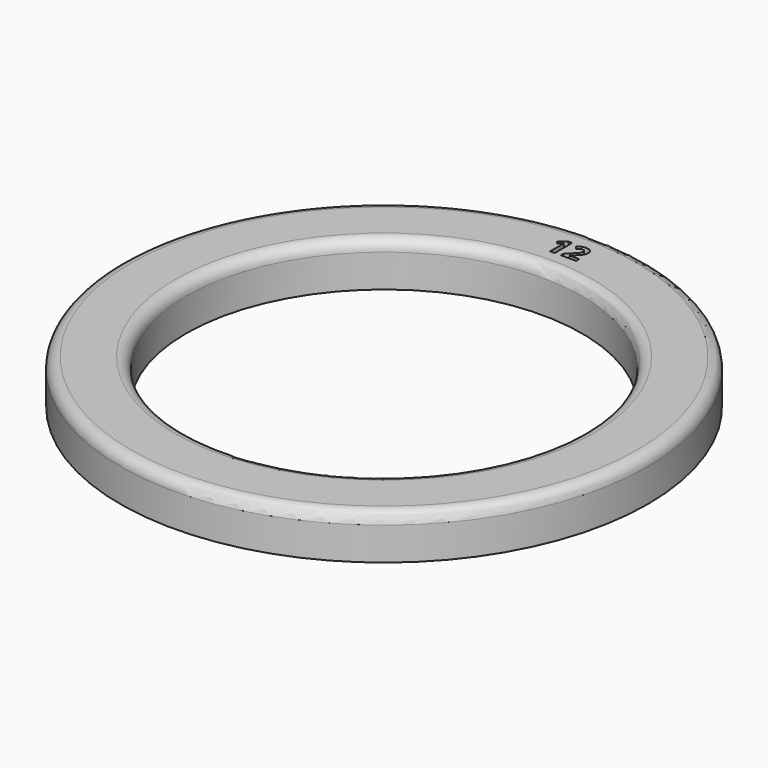
from build123d import *

# Parameters (mm, degrees)
F0_R         = 120
F0_R_2       = 90
F1_DEPTH     = 20
F2_TEXT_SIZE = 13.8888888889
F3_DEPTH     = 25
F4_R         = 5


# Not quite as in the source:
# - Text() gives the source's letters only with a copy of the font that has no kerning and outlines rounded to 1/6400 em; it was checked with that copy


with BuildPart() as f1:
    # F0 (on Top) → F1 (new body)
    with BuildSketch(Plane.XY):
        Circle(F0_R)
        Circle(F0_R_2, mode=Mode.SUBTRACT)
    extrude(amount=F1_DEPTH)

    # F2 (on face) → F3 (cut)
    with BuildSketch(Plane.XY.offset(20)):
        with Locations((-8.1575520833, 100)):
            Text('12', F2_TEXT_SIZE, font='Open Sans', font_style=FontStyle.BOLD, text_align=(TextAlign.LEFT, TextAlign.BOTTOM))
    extrude(amount=-F3_DEPTH, mode=Mode.SUBTRACT)

    # F4
    f4_edges = [f1.edges().sort_by_distance(p)[0] for p in [
        (-90, 0, 20),
        (-120, 0, 20),
    ]]
    fillet(f4_edges, radius=F4_R)


solid = f1.part
